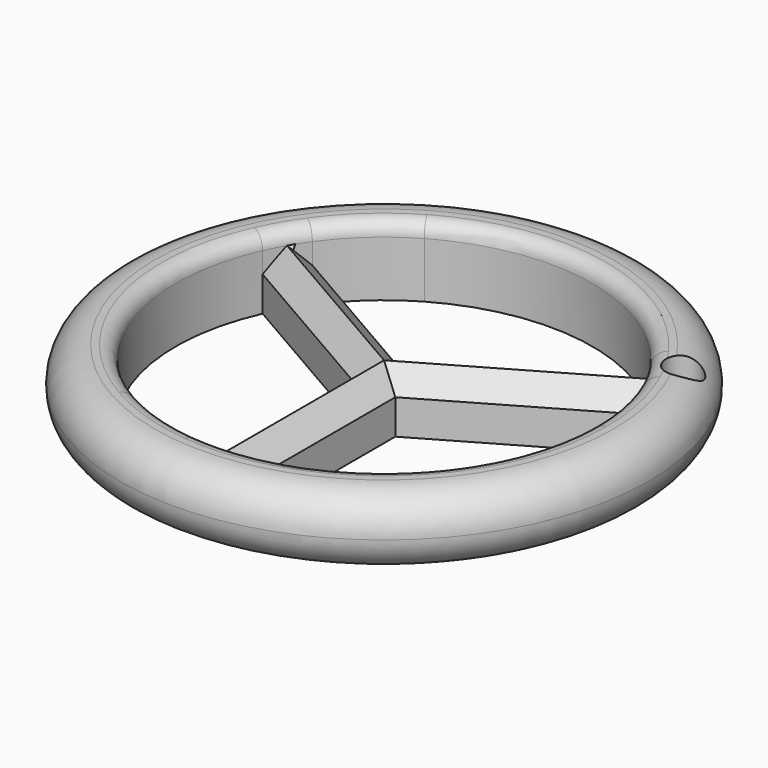
from build123d import *

# Parameters (mm, degrees)
F0_R     = 19
F1_DEPTH = 5
F2_DEPTH = 4
F3_COUNT = 3
F4_SIZE  = 1.4999
F5_R     = 0.99999
F6_R     = 2.49999
F7_R     = 1.25
F8_DEPTH = 5


# Not quite as in the source:
# - a fillet or chamfer is up to 0.001 mm smaller than in the source, because OpenCascade refuses the exact size
# - a feature names something its author has since deleted; it is built from what else it names


with BuildPart() as f1:
    # F0 (on Top) → F1 (new body)
    with BuildSketch(Plane.XY):
        Circle(F0_R)
        with BuildLine():
            ThreePointArc((-1.5, -14.9248115566), (-10.0623058987, 11.1242977306), (15, 0))
            ThreePointArc((15, 0), (11.1242977306, -10.0623058987), (1.5, -14.9248115566))
            ThreePointArc((1.5, -14.9248115566), (0, -15), (-1.5, -14.9248115566))
        make_face(mode=Mode.SUBTRACT)
    extrude(amount=F1_DEPTH)

    # F0 (on Top) → F2 (join)
    with BuildSketch(Plane.XY):
        with BuildLine():
            ThreePointArc((1.5, 0), (0, 1.5), (-1.5, 0))
            ThreePointArc((-1.5, 0), (0, -1.5), (1.5, 0))
        make_face()
        with BuildLine():
            Line((-1.5, 0), (-1.5, -14.9248115566))
            ThreePointArc((-1.5, -14.9248115566), (0, -15), (1.5, -14.9248115566))
            Line((1.5, -14.9248115566), (1.5, 0))
            ThreePointArc((1.5, 0), (0, -1.5), (-1.5, 0))
        make_face()
    extrude(amount=F2_DEPTH)

    # F3: F1 ×3 about axis
    f3_axis = Axis((0, 0, 0), (0, 0, 1))


with BuildPart() as f1_1:
    add(f1.part)
    for i in range(1, F3_COUNT):
        add(f1.part.rotate(f3_axis, i * 360 / F3_COUNT))

    # F4 (size 1.5 in the source; OpenCascade refuses exactly that, so slightly less here)
    f4_edges = [f1_1.edges().sort_by_distance(p)[0] for p in [
        (-7.587633, 2.648671, 4),
        (-6.087633, 5.246747, 4),
        (-1.5, -7.895418, 4),
        (1.5, -7.895418, 4),
        (7.587633, 2.648671, 4),
        (6.087633, 5.246747, 4),
    ]]
    chamfer(f4_edges, length=F4_SIZE)

    # F5 (radius 1 in the source; OpenCascade refuses exactly that, so slightly less here)
    f5_edges = [f1_1.edges().sort_by_distance(p)[0] for p in [
        (-15, 0, 5),
    ]]
    fillet(f5_edges, radius=F5_R)

    # F6 (radius 2.5 in the source; OpenCascade refuses exactly that, so slightly less here)
    f6_edges = [f1_1.edges().sort_by_distance(p)[0] for p in [
        (-19, 0, 5),
        (-19, 0, 0),
    ]]
    fillet(f6_edges, radius=F6_R)

    # F7 (on Top) → F8 (cut)
    with BuildSketch(Plane.XY):
        with Locations((14.7157208627, 8.5116132132)):
            Circle(F7_R)
    extrude(amount=F8_DEPTH, mode=Mode.SUBTRACT)


solid = f1_1.part
